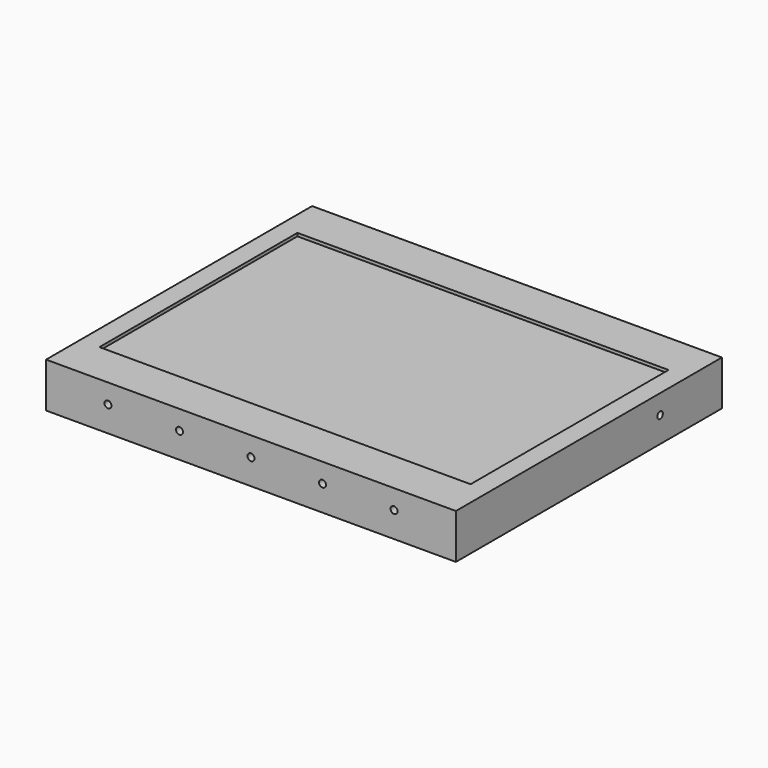
from build123d import *

# Parameters (mm, degrees)
F0_W     = 530
F0_H     = 430
F1_DEPTH = 58
F3_D     = 9
F5_D     = 9
F5_DEPTH = 180
F5_TIP   = 2.7038727856
F7_D     = 9
F7_DEPTH = 180
F7_TIP   = 2.7038727856
F8_W     = 480
F8_H     = 320
F9_DEPTH = 4


# Not quite as in the source:
# - a feature names something its author has since deleted; it is built from what else it names


with BuildPart() as f1:
    # F0 (on Top) → F1 (new body)
    with BuildSketch(Plane.XY):
        with Locations((-265, 215)):
            Rectangle(F0_W, F0_H)
    extrude(amount=F1_DEPTH)

    # F3 (through all)
    with Locations(Plane.XZ):
        with Locations((-450, 33), (-357.5, 33), (-265, 33), (-172.5, 33), (-80, 33)):
            Hole(F3_D / 2)

    # F5
    with Locations(Plane(origin=(-530, 0, 0), x_dir=(0, -1, 0), z_dir=(-1, 0, 0))):
        with Locations((-330, 33)):
            Hole(F5_D / 2, depth=F5_DEPTH)
            with Locations((0, 0, -(F5_DEPTH + F5_TIP / 2))):  # 118° drill point
                Cone(0, F5_D / 2, F5_TIP, mode=Mode.SUBTRACT)

    # F7
    with Locations(Plane.YZ):
        with Locations((330, 33)):
            Hole(F7_D / 2, depth=F7_DEPTH)
            with Locations((0, 0, -(F7_DEPTH + F7_TIP / 2))):  # 118° drill point
                Cone(0, F7_D / 2, F7_TIP, mode=Mode.SUBTRACT)

    # F8 (on face) → F9 (cut)
    with BuildSketch(Plane.XY.offset(58)):
        with Locations((-265, 215)):
            Rectangle(F8_W, F8_H)
    extrude(amount=-F9_DEPTH, mode=Mode.SUBTRACT)


solid = f1.part
